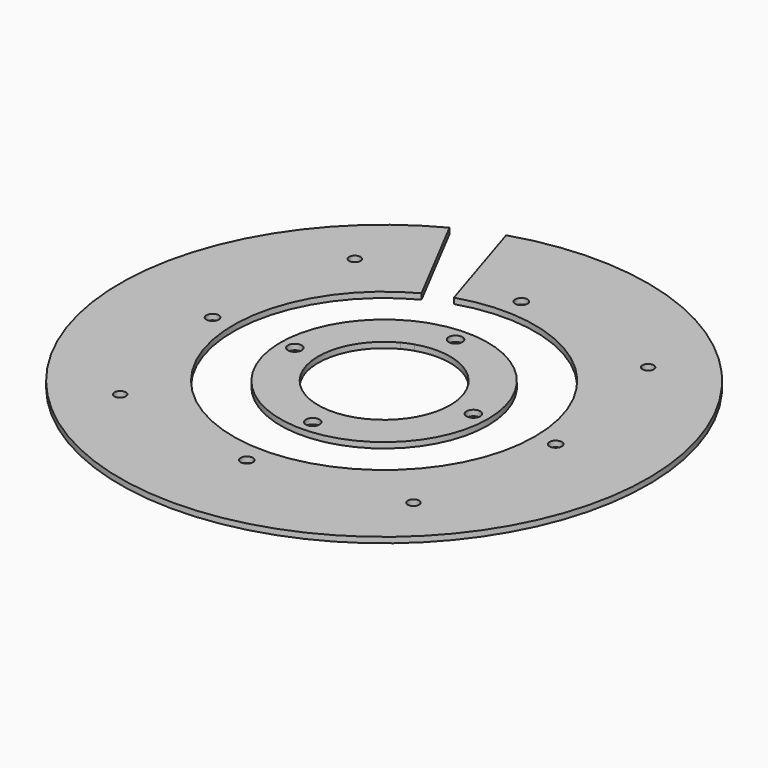
from build123d import *

# Parameters (mm, degrees)
F0_R     = 3
F0_R_2   = 3.25
F1_DEPTH = 3
F0_R_3   = 3.65
F2_DEPTH = 3


# Not quite as in the source:
# - a feature names something its author has since deleted; it is built from what else it names


with BuildPart() as f1:
    # F0 (on Top) → F1 (new body)
    with BuildSketch(Plane.XY):
        with BuildLine():
            ThreePointArc((-24.0564639603, 76.2973560599), (47.3047718691, 64.5155683414), (80, 0))
            ThreePointArc((80, 0), (-41.5018606528, -68.3929496538), (-36.9398890588, 70.9608666543))
            Line((-36.9398890588, 70.9608666543), (-64.6448058529, 124.181516645))
            ThreePointArc((-64.6448058529, 124.181516645), (-72.6282561425, -119.6876618942), (140, 0))
            ThreePointArc((140, 0), (82.7833507709, 112.9022445974), (-42.0988119306, 133.5203731048))
            Line((-42.0988119306, 133.5203731048), (-24.0564639603, 76.2973560599))
        make_face()
        with Locations((-77.7817459305, -77.7817459305)):
            Circle(F0_R, mode=Mode.SUBTRACT)
        with Locations((0, -91)):
            Circle(F0_R_2, mode=Mode.SUBTRACT)
        with Locations((77.7817459305, -77.7817459305)):
            Circle(F0_R, mode=Mode.SUBTRACT)
        with Locations((-91, 0)):
            Circle(F0_R_2, mode=Mode.SUBTRACT)
        with Locations((-77.7817459305, 77.7817459305)):
            Circle(F0_R, mode=Mode.SUBTRACT)
        with Locations((91, 0)):
            Circle(F0_R_2, mode=Mode.SUBTRACT)
        with Locations((0, 91)):
            Circle(F0_R_2, mode=Mode.SUBTRACT)
        with Locations((77.7817459305, 77.7817459305)):
            Circle(F0_R, mode=Mode.SUBTRACT)
    extrude(amount=F1_DEPTH)


with BuildPart() as f2:
    # F0 (on Top) → F2 (new body)
    with BuildSketch(Plane.XY):
        with BuildLine():
            ThreePointArc((55, 0), (32.52203066, 44.3544532347), (-16.5388189727, 52.4544322912))
            Line((-16.5388189727, 52.4544322912), (-10.5247029826, 33.3800932762))
            ThreePointArc((-10.5247029827, 33.3800932762), (20.6958376927, 28.2255611494), (35, 0))
            ThreePointArc((35, 0), (-18.1570640356, -29.9219154736), (-16.1612014632, 31.0453791612))
            Line((-16.1612014632, 31.0453791612), (-25.3961737279, 48.7855958248))
            ThreePointArc((-25.3961737279, 48.7855958248), (-28.5325291988, -47.020152887), (55, 0))
        make_face()
        with Locations((0, -47.35)):
            Circle(F0_R_3, mode=Mode.SUBTRACT)
        with Locations((-47.35, 0)):
            Circle(F0_R_3, mode=Mode.SUBTRACT)
        with Locations((47.35, 0)):
            Circle(F0_R_3, mode=Mode.SUBTRACT)
        with Locations((0, 47.35)):
            Circle(F0_R_3, mode=Mode.SUBTRACT)
        with BuildLine():
            Line((-10.5247029826, 33.3800932762), (-16.5388189727, 52.4544322912))
            ThreePointArc((-16.5388189727, 52.4544322912), (-21.0475887801, 50.8133742881), (-25.3961737279, 48.7855958248))
            Line((-25.3961737279, 48.7855958248), (-16.1612014632, 31.0453791612))
            ThreePointArc((-16.1612014632, 31.0453791612), (-13.3939201328, 32.3357836379), (-10.5247029827, 33.3800932762))
        make_face()
    extrude(amount=F2_DEPTH)


solid = Compound([f1.part, f2.part])
